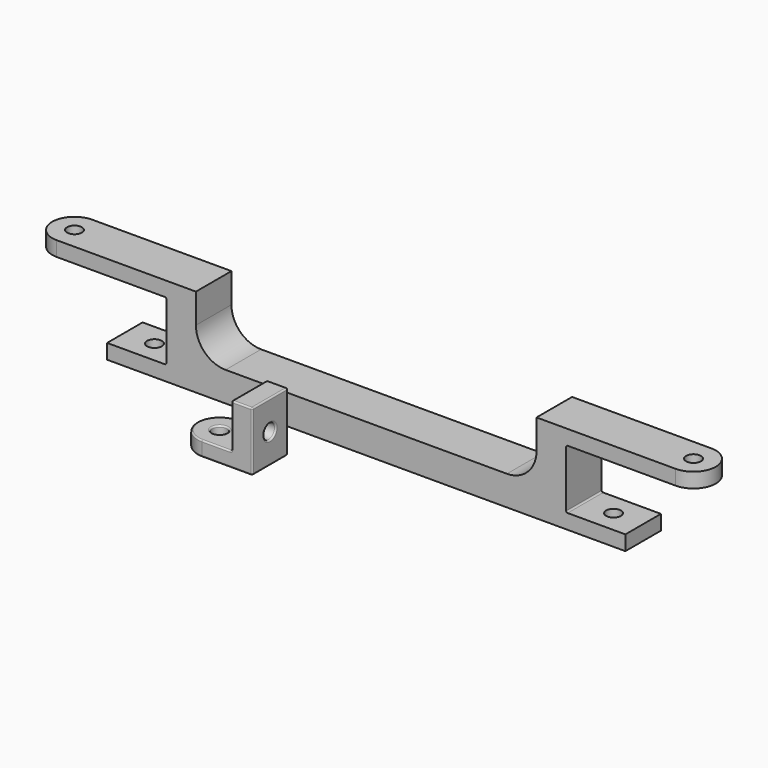
from build123d import *

# Parameters (mm, degrees)
F0_R          = 2.5
F1_DEPTH      = 30
F3_DEPTH      = 25
F4_R          = 2.5
F5_DEPTH      = 25
F6_W          = 7
F6_H          = 15
F7_DEPTH      = 20
F6_R          = 2.5
F8_DEPTH      = 5
F9_R          = 4.5
F9_R_2        = 2.5
F10_DEPTH     = 3
F11_DEPTH     = 7
F12_T1_DEPTH  = 15
F12_T3_DEPTH  = 7.75
F12_T5_DEPTH  = 17.5
F12_T7_DEPTH  = 14
F12_T9_DEPTH  = 19
F12_T11_DEPTH = 16.5
F12_S15_W     = 0.5
F12_S15_H     = 0.5
F12_T16_DEPTH = 0.5
F12_S21_W     = 0.5
F12_S21_H     = 0.5
F12_T22_DEPTH = 0.5
F12_S27_W     = 0.5
F12_S27_H     = 0.5
F12_T28_DEPTH = 0.5
F12_S33_W     = 0.5
F12_S33_H     = 0.5
F12_T34_DEPTH = 0.5
F12_T40_ANGLE = 180
F12_T45_DEPTH = 14
F12_T47_DEPTH = 9.5
F12_S51_W     = 0.5
F12_S51_H     = 0.5
F12_T52_DEPTH = 0.5
F12_S57_W     = 0.5
F12_S57_H     = 0.5
F12_T58_DEPTH = 0.5
F12_T62_ANGLE = 180
F12_T64_ANGLE = 90
F12_T66_ANGLE = 90


# Not quite as in the source:
# - a fillet or chamfer that OpenCascade refuses, or shapes differently, is made with other operations: its cross-section is extruded or revolved along the edge and cut away or added


with BuildPart() as f1:
    # F0 (on Top) → F1 (new body)
    with BuildSketch(Plane.XY):
        with BuildLine():
            ThreePointArc((-97, 0), (-99.1966991411, 5.3033008589), (-104.5, 7.5))
            ThreePointArc((-104.5, 7.5), (-112, 0), (-104.5, -7.5))
            ThreePointArc((-104.5, -7.5), (-99.1966991411, -5.3033008589), (-97, 0))
        make_face()
        with Locations((-104.5, 0)):
            Circle(F0_R, mode=Mode.SUBTRACT)
        with BuildLine():
            ThreePointArc((104.5, -7.5), (97, 0), (104.5, 7.5))
            Line((104.5, 7.5), (-104.5, 7.5))
            ThreePointArc((-104.5, 7.5), (-99.1966991411, 5.3033008589), (-97, 0))
            ThreePointArc((-97, 0), (-99.1966991411, -5.3033008589), (-104.5, -7.5))
            Line((-104.5, -7.5), (104.5, -7.5))
        make_face()
        with BuildLine():
            ThreePointArc((104.5, -7.5), (109.8033008589, -5.3033008589), (112, 0))
            ThreePointArc((112, 0), (109.8033008589, 5.3033008589), (104.5, 7.5))
            ThreePointArc((104.5, 7.5), (97, 0), (104.5, -7.5))
        make_face()
        with Locations((104.5, 0)):
            Circle(F0_R, mode=Mode.SUBTRACT)
    extrude(amount=F1_DEPTH)

    # F2 (on face) → F3 (cut)
    with BuildSketch(Plane.XZ.offset(7.5)):
        with BuildLine():
            Line((57.5, 30), (0, 30))
            Line((0, 30), (0, 10))
            Line((0, 10), (47.5, 10))
            ThreePointArc((47.5, 10), (54.5710678119, 12.9289321881), (57.5, 20))
            Line((57.5, 20), (57.5, 30))
        make_face()
        with BuildLine():
            Line((0, 10), (0, 30))
            Line((0, 30), (-57.5, 30))
            Line((-57.5, 30), (-57.5, 20))
            ThreePointArc((-57.5, 20), (-54.5710678119, 12.9289321881), (-47.5, 10))
            Line((-47.5, 10), (0, 10))
        make_face()
        with BuildLine():
            Line((104.5, 0), (104.5, 25))
            Line((104.5, 25), (68, 25))
            ThreePointArc((68, 25), (67.6464466094, 24.8535533906), (67.5, 24.5))
            Line((67.5, 24.5), (67.5, 5.5))
            ThreePointArc((67.5, 5.5), (67.6464466094, 5.1464466094), (68, 5))
            Line((68, 5), (87.5, 5))
            Line((87.5, 5), (87.5, 0))
            Line((87.5, 0), (104.5, 0))
        make_face()
        Polygon((118.8175827265, 25), (104.5, 25), (104.5, 0), (118.8175827265, 0), (118.8175827265, 5), align=None)
        with BuildLine():
            Line((-68, 25), (-104.5, 25))
            Line((-104.5, 25), (-104.5, 0))
            Line((-104.5, 0), (-87.5, 0))
            Line((-87.5, 0), (-87.5, 5))
            Line((-87.5, 5), (-68, 5))
            ThreePointArc((-68, 5), (-67.6464466094, 5.1464466094), (-67.5, 5.5))
            Line((-67.5, 5.5), (-67.5, 24.5))
            ThreePointArc((-67.5, 24.5), (-67.6464466094, 24.8535533906), (-68, 25))
        make_face()
        Polygon((-104.5, 0), (-104.5, 25), (-118.8175827265, 25), (-118.8175827265, 5), (-118.8175827265, 0), align=None)
    extrude(amount=-F3_DEPTH, mode=Mode.SUBTRACT)

    # F4 (on face) → F5 (cut)
    with BuildSketch(Plane(origin=(0, 0, 0), x_dir=(1, 0, 0), z_dir=(0, 0, -1))):
        with Locations((-77.5, 0)):
            Circle(F4_R)
        with Locations((77.5, 0)):
            Circle(F4_R)
    extrude(amount=-F5_DEPTH, mode=Mode.SUBTRACT)


with BuildPart() as f7:
    # F6 (on Top) → F7 (new body)
    with BuildSketch(Plane.XY):
        with Locations((-19.7659818232, -27.7775004506)):
            Rectangle(F6_W, F6_H)
    extrude(amount=F7_DEPTH)

    # F6 (on Top) → F8 (join)
    with BuildSketch(Plane.XY):
        with BuildLine():
            ThreePointArc((-33.2659818232, -35.2775004506), (-27.9626809643, -33.0808013095), (-25.7659818232, -27.7775004506))
            ThreePointArc((-25.7659818232, -27.7775004506), (-27.9626809643, -22.4741995917), (-33.2659818232, -20.2775004506))
            ThreePointArc((-33.2659818232, -20.2775004506), (-40.7659818232, -27.7775004506), (-33.2659818232, -35.2775004506))
        make_face()
        with Locations((-33.2659818232, -27.7775004506)):
            Circle(F6_R, mode=Mode.SUBTRACT)
        with BuildLine():
            Line((-25.7659818232, -35.2775004506), (-25.7659818232, -27.7775004506))
            ThreePointArc((-25.7659818232, -27.7775004506), (-27.9626809643, -33.0808013095), (-33.2659818232, -35.2775004506))
            Line((-33.2659818232, -35.2775004506), (-25.7659818232, -35.2775004506))
        make_face()
        with BuildLine():
            ThreePointArc((-33.2659818232, -20.2775004506), (-27.9626809643, -22.4741995917), (-25.7659818232, -27.7775004506))
            Line((-25.7659818232, -27.7775004506), (-25.7659818232, -20.2775004506))
            Line((-25.7659818232, -20.2775004506), (-33.2659818232, -20.2775004506))
        make_face()
        Polygon((-25.7659818232, -20.2775004506), (-25.7659818232, -27.7775004506), (-25.7659818232, -35.2775004506), (-23.2659818232, -35.2775004506), (-23.2659818232, -20.2775004506), align=None)
    extrude(amount=F8_DEPTH)

    # F9 (on face) → F10 (cut)
    with BuildSketch(Plane(origin=(-23.2659818232, 0, 0), x_dir=(0, -1, 0), z_dir=(-1, 0, 0))):
        with Locations((27.7775004506, 10)):
            Circle(F9_R)
        with Locations((27.7775004506, 10)):
            Circle(F9_R_2, mode=Mode.SUBTRACT)
    extrude(amount=-F10_DEPTH, mode=Mode.SUBTRACT)

    # F11 (cut, through all): a face of the model
    f11_faces = [f7.faces().sort_by_distance(p)[0] for p in [
        (-23.2659818232, -27.7775004506, 10),
    ]]
    extrude(f11_faces, amount=-F11_DEPTH, mode=Mode.SUBTRACT)

    # F12: fillet of radius 0.5 on 20 edges, made by hand

    # F12_s2 → F12_t1 (join)
    with BuildSketch(Plane.XZ.offset(20.2775004506)):
        with BuildLine():
            ThreePointArc((-23.2659818232, 5.5), (-23.4124284326, 5.1464466094), (-23.7659818232, 5))
            Line((-23.7659818232, 5), (-23.2659818232, 5))
            Line((-23.2659818232, 5), (-23.2659818232, 5.5))
        make_face()
    extrude(amount=F12_T1_DEPTH)

    # F12_s4 → F12_t3 (cut)
    with BuildSketch(Plane.YZ.offset(-24.5159818232)):
        with BuildLine():
            ThreePointArc((-20.2775004506, 19.5), (-20.42394706, 19.8535533906), (-20.7775004506, 20))
            Line((-20.7775004506, 20), (-20.2775004506, 20))
            Line((-20.2775004506, 20), (-20.2775004506, 19.5))
        make_face()
        with BuildLine():
            ThreePointArc((-34.7775004506, 20), (-35.1310538412, 19.8535533906), (-35.2775004506, 19.5))
            Line((-35.2775004506, 19.5), (-35.2775004506, 20))
            Line((-35.2775004506, 20), (-34.7775004506, 20))
        make_face()
    extrude(amount=F12_T3_DEPTH, mode=Mode.SUBTRACT)

    # F12_s6 → F12_t5 (cut)
    with BuildSketch(Plane.XZ.offset(19.0275004506)):
        with BuildLine():
            ThreePointArc((-22.7659818232, 20), (-23.1195352138, 19.8535533906), (-23.2659818232, 19.5))
            Line((-23.2659818232, 19.5), (-23.2659818232, 20))
            Line((-23.2659818232, 20), (-22.7659818232, 20))
        make_face()
    extrude(amount=F12_T5_DEPTH, mode=Mode.SUBTRACT)

    # F12_s8 → F12_t7 (cut)
    with BuildSketch(Plane.XZ.offset(20.7775004506)):
        with BuildLine():
            ThreePointArc((-16.2659818232, 19.5), (-16.4124284326, 19.8535533906), (-16.7659818232, 20))
            Line((-16.7659818232, 20), (-16.2659818232, 20))
            Line((-16.2659818232, 20), (-16.2659818232, 19.5))
        make_face()
        with BuildLine():
            ThreePointArc((-16.2659818232, 0.5), (-16.4124284326, 0.1464466094), (-16.7659818232, 0))
            Line((-16.7659818232, 0), (-16.2659818232, 0))
            Line((-16.2659818232, 0), (-16.2659818232, 0.5))
        make_face()
    extrude(amount=F12_T7_DEPTH, mode=Mode.SUBTRACT)

    # F12_s10 → F12_t9 (cut)
    with BuildSketch(Plane.XY.offset(0.5)):
        with BuildLine():
            ThreePointArc((-16.2659818232, -34.7775004506), (-16.4124284326, -35.1310538412), (-16.7659818232, -35.2775004506))
            Line((-16.7659818232, -35.2775004506), (-16.2659818232, -35.2775004506))
            Line((-16.2659818232, -35.2775004506), (-16.2659818232, -34.7775004506))
        make_face()
        with BuildLine():
            ThreePointArc((-16.7659818232, -20.2775004506), (-16.4124284326, -20.42394706), (-16.2659818232, -20.7775004506))
            Line((-16.2659818232, -20.7775004506), (-16.2659818232, -20.2775004506))
            Line((-16.2659818232, -20.2775004506), (-16.7659818232, -20.2775004506))
        make_face()
    extrude(amount=F12_T9_DEPTH, mode=Mode.SUBTRACT)

    # F12_s12 → F12_t11 (cut)
    with BuildSketch(Plane.YZ.offset(-33.2659818232)):
        with BuildLine():
            ThreePointArc((-34.7775004506, 0), (-35.1310538412, 0.1464466094), (-35.2775004506, 0.5))
            Line((-35.2775004506, 0.5), (-35.2775004506, 0))
            Line((-35.2775004506, 0), (-34.7775004506, 0))
        make_face()
        with BuildLine():
            ThreePointArc((-20.2775004506, 0.5), (-20.42394706, 0.1464466094), (-20.7775004506, 0))
            Line((-20.7775004506, 0), (-20.2775004506, 0))
            Line((-20.2775004506, 0), (-20.2775004506, 0.5))
        make_face()
    extrude(amount=F12_T11_DEPTH, mode=Mode.SUBTRACT)


with BuildPart() as f12_tool14:
    # F12_s15 → F12_t16 (new body)
    with BuildSketch(Plane.XZ.offset(20.7775004506)):
        with Locations((-16.5159818232, 19.75)):
            Rectangle(F12_S15_W, F12_S15_H)
    extrude(amount=-F12_T16_DEPTH)

    # F12_s17 → F12_t18 (revolve, cut)
    with BuildSketch(Plane(origin=(-16.7659818232, -20.7775004506, 19.5), x_dir=(-0.7071067812, 0, -0.7071067812), z_dir=(0.7071067812, 0, -0.7071067812))):
        with BuildLine():
            ThreePointArc((0, -0.5), (0.5, 0), (0, 0.5))
            Line((0, 0.5), (0, -0.5))
        make_face()
    revolve(axis=Axis((-16.7659818232, -20.7775004506, 19.5), (0, 1, 0)), mode=Mode.SUBTRACT)


with BuildPart() as f7_1:
    add(f7.part)

    # F12_t13: cut F12_tool14
    add(f12_tool14.part, mode=Mode.SUBTRACT)


with BuildPart() as f12_tool20:
    # F12_s21 → F12_t22 (new body)
    with BuildSketch(Plane.YZ.offset(-16.7659818232)):
        with Locations((-35.0275004506, 19.75)):
            Rectangle(F12_S21_W, F12_S21_H)
    extrude(amount=F12_T22_DEPTH)

    # F12_s23 → F12_t24 (revolve, cut)
    with BuildSketch(Plane(origin=(-16.7659818232, -34.7775004506, 19.5), x_dir=(0, 0.7071067812, -0.7071067812), z_dir=(0, -0.7071067812, -0.7071067812))):
        with BuildLine():
            ThreePointArc((0, -0.5), (0.5, 0), (0, 0.5))
            Line((0, 0.5), (0, -0.5))
        make_face()
    revolve(axis=Axis((-16.7659818232, -34.7775004506, 19.5), (1, 0, 0)), mode=Mode.SUBTRACT)


with BuildPart() as f7_2:
    add(f7_1.part)

    # F12_t19: cut F12_tool20
    add(f12_tool20.part, mode=Mode.SUBTRACT)


with BuildPart() as f12_tool26:
    # F12_s27 → F12_t28 (new body)
    with BuildSketch(Plane.YZ.offset(-16.7659818232)):
        with Locations((-35.0275004506, 0.25)):
            Rectangle(F12_S27_W, F12_S27_H)
    extrude(amount=F12_T28_DEPTH)

    # F12_s29 → F12_t30 (revolve, cut)
    with BuildSketch(Plane(origin=(-16.7659818232, -34.7775004506, 0.5), x_dir=(0, 0.7071067812, 0.7071067812), z_dir=(0, 0.7071067812, -0.7071067812))):
        with BuildLine():
            ThreePointArc((0, -0.5), (0.5, 0), (0, 0.5))
            Line((0, 0.5), (0, -0.5))
        make_face()
    revolve(axis=Axis((-16.7659818232, -34.7775004506, 0.5), (1, 0, 0)), mode=Mode.SUBTRACT)


with BuildPart() as f7_3:
    add(f7_2.part)

    # F12_t25: cut F12_tool26
    add(f12_tool26.part, mode=Mode.SUBTRACT)


with BuildPart() as f12_tool32:
    # F12_s33 → F12_t34 (new body)
    with BuildSketch(Plane.XZ.offset(20.7775004506)):
        with Locations((-16.5159818232, 0.25)):
            Rectangle(F12_S33_W, F12_S33_H)
    extrude(amount=-F12_T34_DEPTH)

    # F12_s35 → F12_t36 (revolve, cut)
    with BuildSketch(Plane(origin=(-16.7659818232, -20.7775004506, 0.5), x_dir=(-0.7071067812, 0, 0.7071067812), z_dir=(-0.7071067812, 0, -0.7071067812))):
        with BuildLine():
            ThreePointArc((0, -0.5), (0.5, 0), (0, 0.5))
            Line((0, 0.5), (0, -0.5))
        make_face()
    revolve(axis=Axis((-16.7659818232, -20.7775004506, 0.5), (0, 1, 0)), mode=Mode.SUBTRACT)


with BuildPart() as f7_4:
    add(f7_3.part)

    # F12_t31: cut F12_tool32
    add(f12_tool32.part, mode=Mode.SUBTRACT)

    # F12_s37 → F12_t38 (revolve, cut)
    with BuildSketch(Plane.XZ.offset(27.7775004506)):
        with BuildLine():
            ThreePointArc((-30.2659818232, 5), (-30.6195352138, 4.8535533906), (-30.7659818232, 4.5))
            Line((-30.7659818232, 4.5), (-30.7659818232, 5))
            Line((-30.7659818232, 5), (-30.2659818232, 5))
        make_face()
    revolve(axis=Axis((-33.2659818232, -27.7775004506, 5), (0, 0, 1)), mode=Mode.SUBTRACT)

    # F12_s39 → F12_t40 (revolve, cut)
    with BuildSketch(Plane.YZ.offset(-33.2659818232)):
        with BuildLine():
            ThreePointArc((-20.2775004506, 0.5), (-20.42394706, 0.1464466094), (-20.7775004506, 0))
            Line((-20.7775004506, 0), (-20.2775004506, 0))
            Line((-20.2775004506, 0), (-20.2775004506, 0.5))
        make_face()
    revolve(axis=Axis((-33.2659818232, -27.7775004506, 0), (0, 0, 1)), revolution_arc=F12_T40_ANGLE, mode=Mode.SUBTRACT)

    # F12_s41 → F12_t42 (revolve, cut)
    with BuildSketch(Plane.XZ.offset(27.7775004506)):
        with BuildLine():
            ThreePointArc((-30.2659818232, 0), (-30.6195352138, 0.1464466094), (-30.7659818232, 0.5))
            Line((-30.7659818232, 0.5), (-30.7659818232, 0))
            Line((-30.7659818232, 0), (-30.2659818232, 0))
        make_face()
    revolve(axis=Axis((-33.2659818232, -27.7775004506, 0), (0, 0, 1)), mode=Mode.SUBTRACT)

    # F12_s43 → F12_t44 (revolve, cut)
    with BuildSketch(Plane.XY.offset(10)):
        with BuildLine():
            ThreePointArc((-16.2659818232, -30.7775004506), (-16.4124284326, -30.42394706), (-16.7659818232, -30.2775004506))
            Line((-16.7659818232, -30.2775004506), (-16.2659818232, -30.2775004506))
            Line((-16.2659818232, -30.2775004506), (-16.2659818232, -30.7775004506))
        make_face()
    revolve(axis=Axis((-16.2659818232, -27.7775004506, 10), (-1, 0, 0)), mode=Mode.SUBTRACT)

    # F12_s46 → F12_t45 (cut)
    with BuildSketch(Plane.XY.offset(5.5)):
        with BuildLine():
            ThreePointArc((-23.2659818232, -34.7775004506), (-23.1195352138, -35.1310538412), (-22.7659818232, -35.2775004506))
            Line((-22.7659818232, -35.2775004506), (-23.2659818232, -35.2775004506))
            Line((-23.2659818232, -35.2775004506), (-23.2659818232, -34.7775004506))
        make_face()
        with BuildLine():
            ThreePointArc((-22.7659818232, -20.2775004506), (-23.1195352138, -20.42394706), (-23.2659818232, -20.7775004506))
            Line((-23.2659818232, -20.7775004506), (-23.2659818232, -20.2775004506))
            Line((-23.2659818232, -20.2775004506), (-22.7659818232, -20.2775004506))
        make_face()
    extrude(amount=F12_T45_DEPTH, mode=Mode.SUBTRACT)

    # F12_s48 → F12_t47 (cut)
    with BuildSketch(Plane.YZ.offset(-33.2659818232)):
        with BuildLine():
            ThreePointArc((-34.7775004506, 5), (-35.1310538412, 4.8535533906), (-35.2775004506, 4.5))
            Line((-35.2775004506, 4.5), (-35.2775004506, 5))
            Line((-35.2775004506, 5), (-34.7775004506, 5))
        make_face()
        with BuildLine():
            ThreePointArc((-20.2775004506, 4.5), (-20.42394706, 4.8535533906), (-20.7775004506, 5))
            Line((-20.7775004506, 5), (-20.2775004506, 5))
            Line((-20.2775004506, 5), (-20.2775004506, 4.5))
        make_face()
    extrude(amount=F12_T47_DEPTH, mode=Mode.SUBTRACT)


with BuildPart() as f12_tool50:
    # F12_s51 → F12_t52 (new body)
    with BuildSketch(Plane.XZ.offset(20.7775004506)):
        with Locations((-23.0159818232, 19.75)):
            Rectangle(F12_S51_W, F12_S51_H)
    extrude(amount=-F12_T52_DEPTH)

    # F12_s53 → F12_t54 (revolve, cut)
    with BuildSketch(Plane(origin=(-22.7659818232, -20.7775004506, 19.5), x_dir=(0.7071067812, 0, -0.7071067812), z_dir=(0.7071067812, 0, 0.7071067812))):
        with BuildLine():
            ThreePointArc((0, -0.5), (0.5, 0), (0, 0.5))
            Line((0, 0.5), (0, -0.5))
        make_face()
    revolve(axis=Axis((-22.7659818232, -20.7775004506, 19.5), (0, 1, 0)), mode=Mode.SUBTRACT)


with BuildPart() as f7_5:
    add(f7_4.part)

    # F12_t49: cut F12_tool50
    add(f12_tool50.part, mode=Mode.SUBTRACT)


with BuildPart() as f12_tool56:
    # F12_s57 → F12_t58 (new body)
    with BuildSketch(Plane.YZ.offset(-22.7659818232)):
        with Locations((-35.0275004506, 19.75)):
            Rectangle(F12_S57_W, F12_S57_H)
    extrude(amount=-F12_T58_DEPTH)

    # F12_s59 → F12_t60 (revolve, cut)
    with BuildSketch(Plane(origin=(-22.7659818232, -34.7775004506, 19.5), x_dir=(0, 0.7071067812, -0.7071067812), z_dir=(0, 0.7071067812, 0.7071067812))):
        with BuildLine():
            ThreePointArc((0, -0.5), (0.5, 0), (0, 0.5))
            Line((0, 0.5), (0, -0.5))
        make_face()
    revolve(axis=Axis((-22.7659818232, -34.7775004506, 19.5), (-1, 0, 0)), mode=Mode.SUBTRACT)


with BuildPart() as f7_6:
    add(f7_5.part)

    # F12_t55: cut F12_tool56
    add(f12_tool56.part, mode=Mode.SUBTRACT)

    # F12_s61 → F12_t62 (revolve, cut)
    with BuildSketch(Plane.YZ.offset(-33.2659818232)):
        with BuildLine():
            ThreePointArc((-20.2775004506, 4.5), (-20.42394706, 4.8535533906), (-20.7775004506, 5))
            Line((-20.7775004506, 5), (-20.2775004506, 5))
            Line((-20.2775004506, 5), (-20.2775004506, 4.5))
        make_face()
    revolve(axis=Axis((-33.2659818232, -27.7775004506, 5), (0, 0, 1)), revolution_arc=F12_T62_ANGLE, mode=Mode.SUBTRACT)

    # F12_s63 → F12_t64 (revolve, cut)
    with BuildSketch(Plane.XY.offset(5.5)):
        with BuildLine():
            ThreePointArc((-22.7659818232, -20.2775004506), (-23.1195352138, -20.42394706), (-23.2659818232, -20.7775004506))
            Line((-23.2659818232, -20.7775004506), (-23.2659818232, -20.2775004506))
            Line((-23.2659818232, -20.2775004506), (-22.7659818232, -20.2775004506))
        make_face()
    revolve(axis=Axis((-23.7659818232, -20.2775004506, 5.5), (0, 1, 0)), revolution_arc=F12_T64_ANGLE, mode=Mode.SUBTRACT)

    # F12_s65 → F12_t66 (revolve, cut)
    with BuildSketch(Plane.XY.offset(5.5)):
        with BuildLine():
            ThreePointArc((-23.2659818232, -34.7775004506), (-23.1195352138, -35.1310538412), (-22.7659818232, -35.2775004506))
            Line((-22.7659818232, -35.2775004506), (-23.2659818232, -35.2775004506))
            Line((-23.2659818232, -35.2775004506), (-23.2659818232, -34.7775004506))
        make_face()
    revolve(axis=Axis((-23.7659818232, -35.2775004506, 5.5), (0, 1, 0)), revolution_arc=F12_T66_ANGLE, mode=Mode.SUBTRACT)


solid = Compound([f1.part, f7_6.part])
